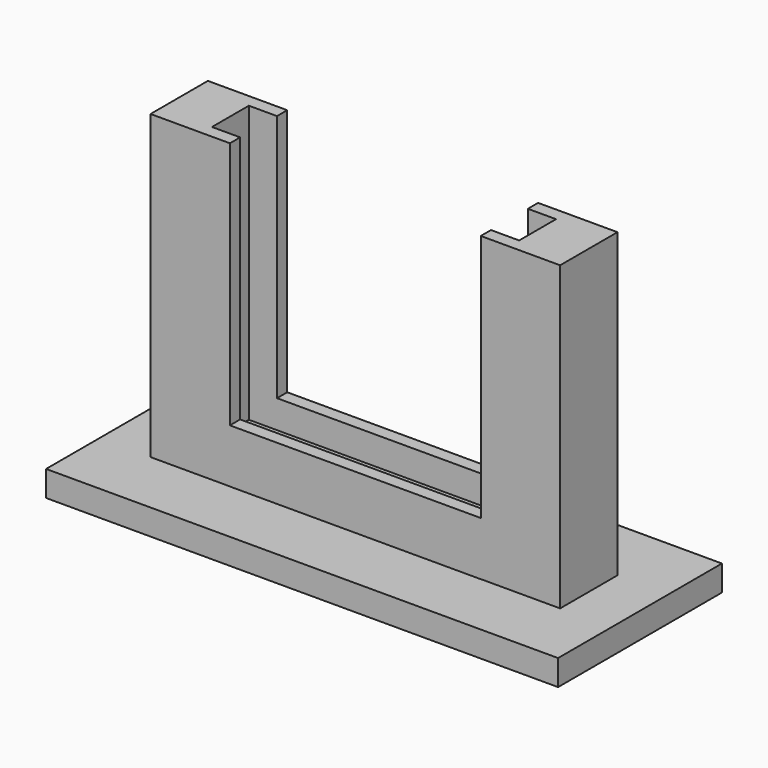
from build123d import *

# Parameters (mm, degrees)
F0_W     = 200
F0_H     = 80
F0_W_2   = 98
F0_H_2   = 18
F0_H_3   = 5
F0_W_3   = 11
F1_DEPTH = 10
F2_DEPTH = 20
F3_DEPTH = 31
F4_DEPTH = 128


# Not quite as in the source:
# - a feature names something its author has since deleted; it is built from what else it names


with BuildPart() as f1:
    # F0 (on Top) → F1 (new body)
    with BuildSketch(Plane.XY):
        Rectangle(F0_W, F0_H)
        Polygon((80, 14), (80, -14), (49, -14), (49, -14.0508310869), (-49, -14.0508310869), (-49, -14), (-80, -14), (-80, 14), (-49, 14), (-49, 14.0508310869), (49, 14.0508310869), (49, 14), align=None, mode=Mode.SUBTRACT)
        Rectangle(F0_W_2, F0_H_2)
        Polygon((49, -14), (80, -14), (80, 14), (49, 14), (49, 9), (60, 9), (60, -9), (49, -9), align=None)
        Polygon((-80, -14), (-49, -14), (-49, -9), (-60, -9), (-60, 9), (-49, 9), (-49, 14), (-80, 14), align=None)
        with Locations((0, -11.5)):
            Rectangle(F0_W_2, F0_H_3)
        with Locations((0, 11.5)):
            Rectangle(F0_W_2, F0_H_3)
        with Locations((54.5, 0)):
            Rectangle(F0_W_3, F0_H_2)
        with Locations((-54.5, 0)):
            Rectangle(F0_W_3, F0_H_2)
    extrude(amount=F1_DEPTH)

    # F0 (on Top) → F2 (join)
    with BuildSketch(Plane.XY):
        Polygon((-80, -14), (-49, -14), (-49, -9), (-60, -9), (-60, 9), (-49, 9), (-49, 14), (-80, 14), align=None)
        with Locations((-54.5, 0)):
            Rectangle(F0_W_3, F0_H_2)
        Rectangle(F0_W_2, F0_H_2)
        with Locations((54.5, 0)):
            Rectangle(F0_W_3, F0_H_2)
        Polygon((49, -14), (80, -14), (80, 14), (49, 14), (49, 9), (60, 9), (60, -9), (49, -9), align=None)
        with Locations((0, -11.5)):
            Rectangle(F0_W_2, F0_H_3)
        with Locations((0, 11.5)):
            Rectangle(F0_W_2, F0_H_3)
    extrude(amount=F2_DEPTH)

    # F0 (on Top) → F3 (join)
    with BuildSketch(Plane.XY):
        Polygon((-80, -14), (-49, -14), (-49, -9), (-60, -9), (-60, 9), (-49, 9), (-49, 14), (-80, 14), align=None)
        with Locations((0, 11.5)):
            Rectangle(F0_W_2, F0_H_3)
        with Locations((0, -11.5)):
            Rectangle(F0_W_2, F0_H_3)
        Polygon((49, -14), (80, -14), (80, 14), (49, 14), (49, 9), (60, 9), (60, -9), (49, -9), align=None)
    extrude(amount=F3_DEPTH)

    # F0 (on Top) → F4 (join)
    with BuildSketch(Plane.XY):
        Polygon((-80, -14), (-49, -14), (-49, -9), (-60, -9), (-60, 9), (-49, 9), (-49, 14), (-80, 14), align=None)
        Polygon((49, -14), (80, -14), (80, 14), (49, 14), (49, 9), (60, 9), (60, -9), (49, -9), align=None)
    extrude(amount=F4_DEPTH)


solid = f1.part
